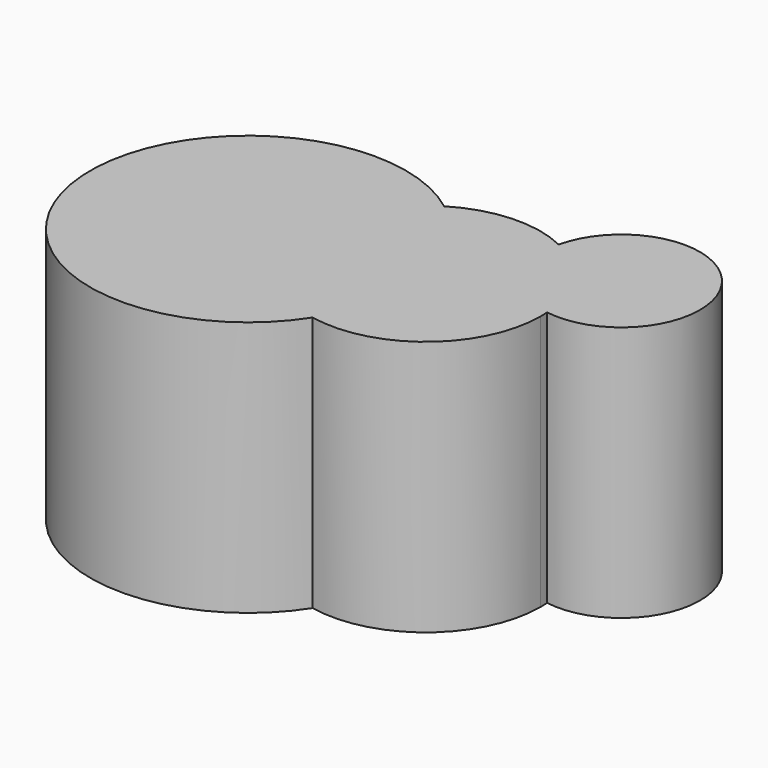
from build123d import *

# Parameters (mm, degrees)
F1_DEPTH = 50.8


# Not quite as in the source:
# - the program builds the solid bodies; features that only make, move or delete a surface that nothing else refers to are left out


with BuildPart() as f1:
    # F0 (on Top) → F1 (new body)
    with BuildSketch(Plane.XY):
        with BuildLine():
            ThreePointArc((71.697641485, 22.5322768092), (57.8335915966, 38.0459789198), (40.8652917128, 26.0058945539))
            ThreePointArc((40.8652917128, 26.0058945539), (49.8001603414, 18.2709960085), (53.6773841191, 7.1073197012))
            ThreePointArc((53.6773841191, 7.1073197012), (66.2378886043, 10.6720599339), (71.697641485, 22.5322768092))
        make_face()
        with BuildLine():
            ThreePointArc((40.8652917128, 26.0058945539), (29.7902072309, 28.2756215729), (18.9821024809, 24.9598971069))
            ThreePointArc((18.9821024809, 24.9598971069), (28.094084627, 13.9297913535), (31.3578806392, 0))
            ThreePointArc((31.3578806392, 0), (30.0861647392, -8.8396475875), (26.3741656765, -16.9623130219))
            ThreePointArc((26.3741656765, -16.9623130219), (45.3624091415, -12.2385728556), (53.7378936923, 5.4452720199))
            ThreePointArc((53.7378936923, 5.4452720199), (53.7227612897, 6.2768464158), (53.6773841191, 7.1073197012))
            ThreePointArc((53.6773841191, 7.1073197012), (43.1635782705, 13.7717941683), (40.8652917128, 26.0058945539))
        make_face()
        with BuildLine():
            ThreePointArc((53.6773841191, 7.1073197012), (49.8001603414, 18.2709960085), (40.8652917128, 26.0058945539))
            ThreePointArc((40.8652917128, 26.0058945539), (43.1635782705, 13.7717941683), (53.6773841191, 7.1073197012))
        make_face()
        with BuildLine():
            ThreePointArc((25.2208191949, -16.6990878355), (28.9640451764, -8.7197099962), (30.2481281305, 0))
            ThreePointArc((30.2481281305, 0), (27.0098398624, 13.6168207012), (17.9883409986, 24.3180764765))
            ThreePointArc((17.9883409986, 24.3180764765), (8.3723071222, 1.4762729148), (25.2208191949, -16.6990878355))
        make_face()
        with BuildLine():
            ThreePointArc((17.9883409986, 24.3180764765), (27.0098398624, 13.6168207012), (30.2481281305, 0))
            ThreePointArc((30.2481281305, 0), (28.9640451764, -8.7197099962), (25.2208191949, -16.6990878355))
            ThreePointArc((25.2208191949, -16.6990878355), (25.7957891487, -16.8381635446), (26.3741656765, -16.9623130219))
            ThreePointArc((26.3741656765, -16.9623130219), (30.0861647392, -8.8396475875), (31.3578806392, 0))
            ThreePointArc((31.3578806392, 0), (28.094084627, 13.9297913535), (18.9821024809, 24.9598971069))
            ThreePointArc((18.9821024809, 24.9598971069), (18.4810686237, 24.6454172593), (17.9883409986, 24.3180764765))
        make_face()
        with BuildLine():
            ThreePointArc((25.2208191949, -16.6990878355), (-29.7885854516, -5.2525643445), (17.9883409986, 24.3180764765))
            ThreePointArc((17.9883409986, 24.3180764765), (18.4810686237, 24.6454172593), (18.9821024809, 24.9598971069))
            ThreePointArc((18.9821024809, 24.9598971069), (-30.881478119, -5.4452720199), (26.3741656765, -16.9623130219))
            ThreePointArc((26.3741656765, -16.9623130219), (25.7957891487, -16.8381635446), (25.2208191949, -16.6990878355))
        make_face()
        with BuildLine():
            ThreePointArc((25.2208191949, -16.6990878355), (8.3723071222, 1.4762729148), (17.9883409986, 24.3180764765))
            ThreePointArc((17.9883409986, 24.3180764765), (-29.7885854516, -5.2525643445), (25.2208191949, -16.6990878355))
        make_face()
    extrude(amount=F1_DEPTH)


solid = f1.part
